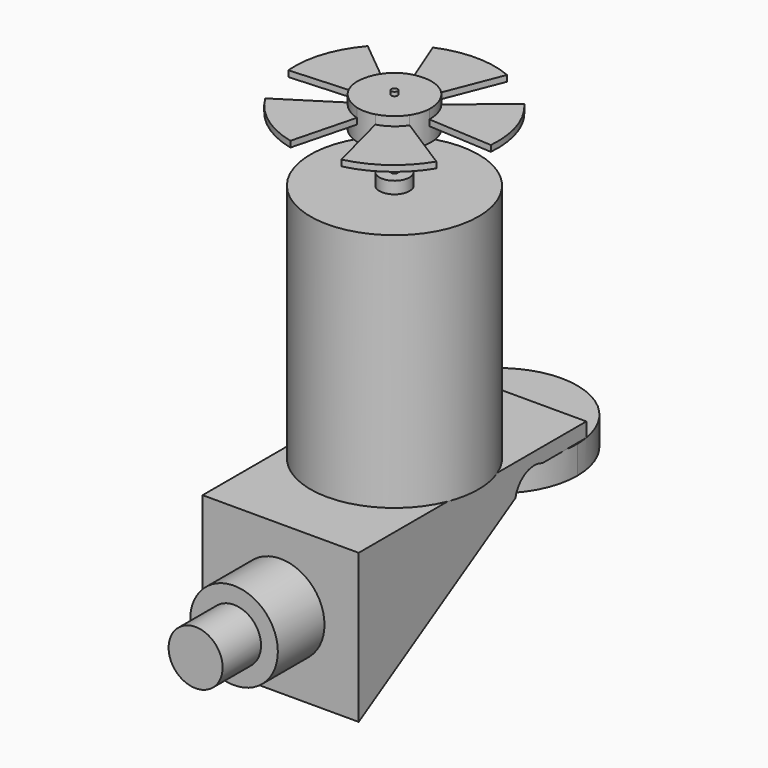
from build123d import *

# Parameters (mm, degrees)
F1_DEPTH  = 50.8
F2_R      = 3.175
F3_DEPTH  = 2.54
F4_R      = 0.635
F5_DEPTH  = 8.0518
F6_R      = 7.7597
F7_DEPTH  = 3.175
F9_DEPTH  = 1.27
F10_DEPTH = 3.175
F11_R     = 0.635
F12_DEPTH = 0.8382
F14_DEPTH = 31.496
F16_DEPTH = 51.816
F18_W     = 26.3473056257
F18_H     = 54.6325752512
F19_DEPTH = 28.448
F21_DEPTH = 5.9436
F22_R     = 9.271
F23_DEPTH = 12.3317
F26_R     = 5.715
F27_DEPTH = 10.16


# Not quite as in the source:
# - a length typed as a fraction of an inch, garbled in the dataset ("3 / 203.2 mm" for 3/8 in), is restored


with BuildPart() as f1:
    # F0 (on Top) → F1 (new body)
    with BuildSketch(Plane.XY):
        with BuildLine():
            Line((0, 35.56), (0, 0))
            ThreePointArc((0, 0), (12.5723585695, 5.2076414305), (17.78, 17.78))
            ThreePointArc((17.78, 17.78), (12.5723585695, 30.3523585695), (0, 35.56))
        make_face()
        with BuildLine():
            ThreePointArc((0, 35.56), (-17.78, 17.78), (0, 0))
            Line((0, 0), (0, 35.56))
        make_face()
    extrude(amount=F1_DEPTH)

    # F2 (on face) → F3 (join)
    with BuildSketch(Plane.XY.offset(50.8)):
        with Locations((0, 17.78)):
            Circle(F2_R)
    extrude(amount=F3_DEPTH)

    # F4 (on face) → F5 (join)
    with BuildSketch(Plane.XY.offset(53.34)):
        with Locations((0, 17.78)):
            Circle(F4_R)
    extrude(amount=F5_DEPTH)

    # F6 (on face) → F7 (join)
    with BuildSketch(Plane.XY.offset(61.3918)):
        with Locations((0, 17.78)):
            Circle(F6_R)
    extrude(amount=F7_DEPTH)

    # F8 (on face) → F9 (join)
    with BuildSketch(Plane.XY.offset(64.5668)):
        with BuildLine():
            Line((-7.8562656417, 37.7526283264), (-2.8404457135, 25.0011364922))
            ThreePointArc((-2.8404457135, 25.0011364922), (0, 25.4905939517), (2.8404457135, 25.0011364922))
            Line((2.8404457135, 25.0011364922), (7.8562656417, 37.7526283264))
            ThreePointArc((7.8562656417, 37.7526283264), (0, 39.3496460261), (-7.8562656417, 37.7526283264))
        make_face()
        with BuildLine():
            ThreePointArc((-7.745454913, 17.3100294897), (-7.3332106223, 20.1627045678), (-5.9899629188, 22.7128782998))
            Line((-5.9899629188, 22.7128782998), (-16.5673787218, 31.4236342075))
            ThreePointArc((-16.5673787218, 31.4236342075), (-20.5139524073, 24.4453871847), (-21.422817913, 16.4801289429))
            Line((-21.422817913, 16.4801289429), (-7.745454913, 17.3100294897))
        make_face()
        with BuildLine():
            ThreePointArc((-1.946508681, 10.2684057588), (-4.5321734112, 11.5419984564), (-6.5424463887, 13.6075499595))
            Line((-6.5424463887, 13.6075499595), (-18.0954687963, 6.2396013439))
            ThreePointArc((-18.0954687963, 6.2396013439), (-12.6783198313, 0.3297898022), (-5.3837639633, -2.9959928207))
            Line((-5.3837639633, -2.9959928207), (-1.946508681, 10.2684057588))
        make_face()
        with BuildLine():
            ThreePointArc((6.5424463887, 13.6075499595), (4.5321734112, 11.5419984564), (1.946508681, 10.2684057588))
            Line((1.946508681, 10.2684057588), (5.3837639633, -2.9959928207))
            ThreePointArc((5.3837639633, -2.9959928207), (12.6783198313, 0.3297898022), (18.0954687963, 6.2396013439))
            Line((18.0954687963, 6.2396013439), (6.5424463887, 13.6075499595))
        make_face()
        with BuildLine():
            ThreePointArc((5.9899629188, 22.7128782998), (7.3332106223, 20.1627045678), (7.745454913, 17.3100294897))
            Line((7.745454913, 17.3100294897), (21.422817913, 16.4801289429))
            ThreePointArc((21.422817913, 16.4801289429), (20.5139524073, 24.4453871847), (16.5673787218, 31.4236342075))
            Line((16.5673787218, 31.4236342075), (5.9899629188, 22.7128782998))
        make_face()
    extrude(amount=F9_DEPTH)

    # F10 (add): a face of the model
    f10_faces = [f1.faces().sort_by_distance(p)[0] for p in [
        (0, 17.78, 64.5668),
    ]]
    extrude(f10_faces, amount=F10_DEPTH)

    # F11 (on face) → F12 (join)
    with BuildSketch(Plane.XY.offset(67.7418)):
        with Locations((0, 17.78)):
            Circle(F11_R)
    extrude(amount=F12_DEPTH)

    # F13 (on face) → F14 (join)
    with BuildSketch(Plane(origin=(0, 0, 0), x_dir=(1, 0, 0), z_dir=(0, 0, -1))):
        with BuildLine():
            Line((-16.51, 12.319), (-16.51, -11.1808864232))
            ThreePointArc((-16.51, -11.1808864232), (0, 0), (16.51, -11.1808864232))
            Line((16.51, -11.1808864232), (16.51, 12.319))
            Line((16.51, 12.319), (-16.51, 12.319))
        make_face()
        with BuildLine():
            ThreePointArc((16.51, -24.3791135768), (0, -35.56), (-16.51, -24.3791135768))
            Line((-16.51, -24.3791135768), (-16.51, -47.879))
            Line((-16.51, -47.879), (16.51, -47.879))
            Line((16.51, -47.879), (16.51, -24.3791135768))
        make_face()
        with BuildLine():
            Line((-16.51, -11.1808864232), (-16.51, -17.78))
            Line((-16.51, -17.78), (-16.51, -24.3791135768))
            ThreePointArc((-16.51, -24.3791135768), (0, -35.56), (16.51, -24.3791135768))
            Line((16.51, -24.3791135768), (16.51, -17.78))
            Line((16.51, -17.78), (16.51, -11.1808864232))
            ThreePointArc((16.51, -11.1808864232), (0, 0), (-16.51, -11.1808864232))
        make_face()
    extrude(amount=F14_DEPTH)

    # F15 (on face) → F16 (cut)
    with BuildSketch(Plane.YZ.offset(16.51)):
        with BuildLine():
            Line((29.1356388479, -6.6541871056), (-12.319, -31.496))
            Line((-12.319, -31.496), (47.879, -31.496))
            Line((47.879, -31.496), (47.879, -3.048))
            Line((47.879, -3.048), (36.2268202007, -3.048))
            ThreePointArc((36.2268202007, -3.048), (31.8141050009, -3.1459858946), (29.1356388479, -6.6541871056))
        make_face()
    extrude(amount=-F16_DEPTH, mode=Mode.SUBTRACT)

    # F18 (on offset) → F19 (cut)
    with BuildSketch(Plane.XY.offset(-31.496)):
        with Locations((0, 17.7540327422)):
            Rectangle(F18_W, F18_H)
    extrude(amount=F19_DEPTH, mode=Mode.SUBTRACT)

    # F20 (on face) → F21 (join)
    with BuildSketch(Plane(origin=(0, 0, -3.048), x_dir=(1, 0, 0), z_dir=(0, 0, -1))):
        with BuildLine():
            ThreePointArc((0, -61.9528820528), (11.813335281, -57.0596383625), (16.7065789713, -45.2463030815))
            ThreePointArc((16.7065789713, -45.2463030815), (-11.813335281, -33.4329678005), (0, -61.9528820528))
        make_face()
    extrude(amount=F21_DEPTH)

    # F22 (on face) → F23 (join)
    with BuildSketch(Plane.XZ.offset(12.319)):
        with Locations((0, -15.748)):
            Circle(F22_R)
    extrude(amount=F23_DEPTH)

    # F26 (on face) → F27 (join)
    with BuildSketch(Plane.XZ.offset(24.6507)):
        with Locations((0, -15.748)):
            Circle(F26_R)
    extrude(amount=F27_DEPTH)


solid = f1.part
